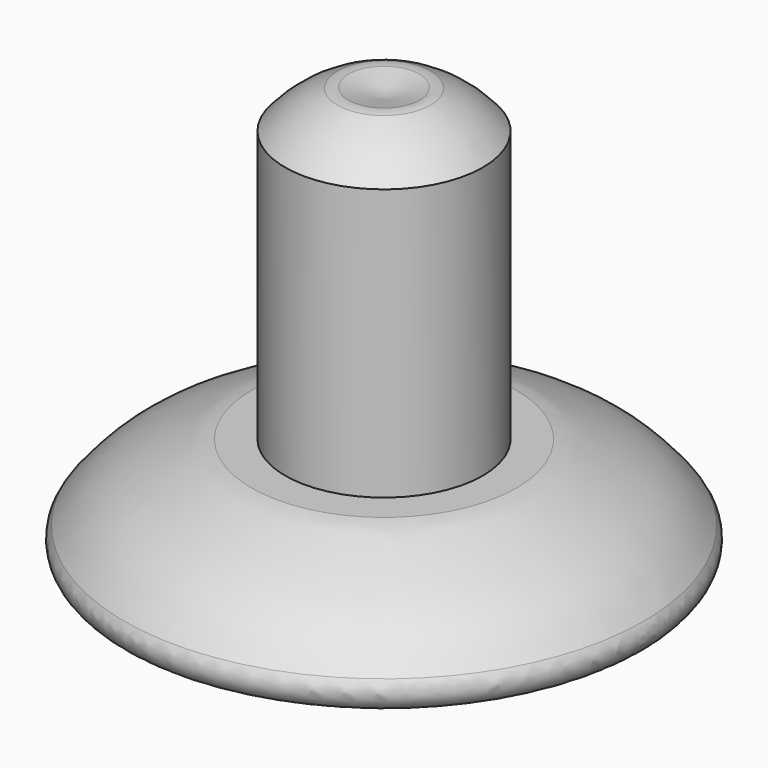
from build123d import *

# Parameters (mm, degrees)
F3_R = 0.762


# Not quite as in the source:
# - a feature names something its author has since deleted; it is built from what else it names


with BuildPart() as f2:
    # F0 (on Front) → F2 (revolve)
    with BuildSketch(Plane.XZ):
        with BuildLine():
            Line((3.8862, 1.0368246978), (3.8862, 11.7048246978))
            ThreePointArc((3.8862, 11.7048246978), (2.8543707216, 12.645076528), (1.6046219265, 13.2670677765))
            Line((1.6046219265, 13.2670677765), (0, 12.9230134189))
            Line((0, 12.9230134189), (0, -0.635))
            add(Edge.make_bspline(
                [(6.0325, -3.175), (4.927107133, -1.9561804365), (4.0449600812, -1.3553717475), (1.9983640724, -0.7115763161), (0.9248232606, -0.5421136513), (0, -0.635)],
                knots=[0, 0, 0, 0, 0.3804425123, 0.6767184943, 1, 1, 1, 1], degree=3))
            Line((6.0325, -3.175), (11.1125, -3.175))
            add(Edge.make_bspline(
                [(5.207, 1.0368246978), (5.7984997261, 0.975644811), (6.74291899, 0.5105425669), (9.2830121982, -0.5417734643), (10.4753485066, -2.2706511595), (11.1125, -3.175)],
                knots=[0, 0, 0, 0, 0.2725407329, 0.6170084006, 1, 1, 1, 1], degree=3))
            Line((5.207, 1.0368246978), (3.8862, 1.0368246978))
        make_face()
    revolve(axis=Axis((0, 0, 1.4091059566), (0, 0, -1)))

    # F3
    f3_edges = [f2.edges().sort_by_distance(p)[0] for p in [
        (-1.604622, 0, 13.267068),
        (-6.0325, 0, -3.175),
        (-11.1125, 0, -3.175),
    ]]
    fillet(f3_edges, radius=F3_R)


solid = f2.part
